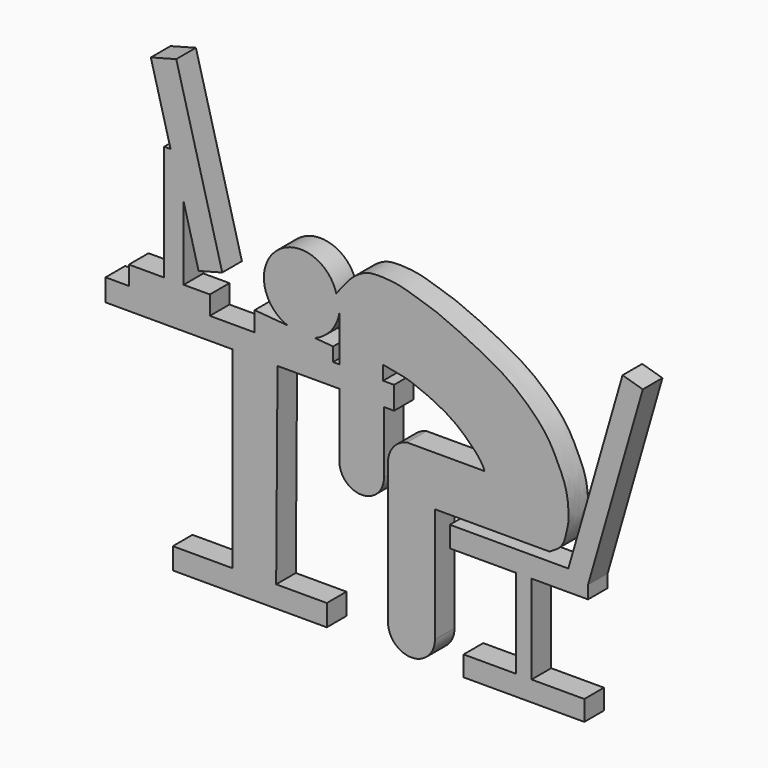
from build123d import *

# Parameters (mm, degrees)
F1_DEPTH = 2


# Not quite as in the source:
# - a feature of the source that left no trace in its solid (it failed there, or was rolled back) is left out


with BuildPart() as f1:
    # F0 (on Front) → F1 (new body)
    with BuildSketch(Plane.XZ):
        with BuildLine():
            Line((18.9171390745, 18.8327007444), (18.9171390745, 19.9865035199))
            add(Edge.make_bspline(
                [(18.9171390745, 19.9865035199), (20.2359017059, 19.7609265773), (20.9778353537, 19.6205597026), (23.2221259054, 18.699726427), (24.7231770067, 17.8086116304), (25.7698344015, 16.9044499376), (26.9919522107, 15.6755559146), (27.1760820528, 15.0417076929)],
                knots=[0, 0, 0, 0, 0.2179321827, 0.4264477532, 0.6140262018, 0.7851447158, 1, 1, 1, 1], degree=3))
            Line((27.1760820528, 15.0417076929), (20.8682008088, 15.0417076929))
            ThreePointArc((20.8682008088, 15.0417076929), (19.753969154, 14.3510608736), (19.318478182, 13.1145929918))
            Line((19.318478182, 13.1145929918), (19.318478182, 1.6501822975))
            ThreePointArc((19.318478182, 1.6501822975), (21.2292131037, -0.2605526242), (23.1399480253, 1.6501822975))
            Line((23.1399480253, 1.6501822975), (23.1399480253, 10.9915547073))
            Line((23.1399480253, 10.9915547073), (32.4813202024, 10.9915547073))
            add(Edge.make_bspline(
                [(32.4813202024, 10.9915547073), (32.7173913015, 11.1297281374), (33.1759580653, 11.3981287793), (33.6647764756, 11.943610763), (33.8785442051, 12.9474288042), (34.0688789671, 13.6968216831), (33.9783273465, 15.2441055836), (33.7191306214, 16.3712863899), (33.0805074051, 17.736024655), (32.5118657998, 18.8903594103), (31.6952000931, 19.9920483371), (30.3992394359, 21.2421100827), (29.0660577632, 22.3165505623), (27.023596623, 23.4836145379), (24.8210679729, 24.5125473654), (23.0257936504, 25.3081835207), (21.5598125958, 25.6984832194), (20.1925631903, 26.2037521602), (18.1718154029, 26.3052282349), (17.4545886694, 26.1074868938), (16.9452981604, 25.8397557796), (16.5052029261, 25.5141227487), (16.0173593733, 25.032961087), (15.6388983087, 24.5073680239), (15.2971428532, 24.1187135914), (15.2342961271, 24.0202073944), (15.1027834162, 23.8599643513)],
                knots=[0, 0, 0, 0, 0.0347440285, 0.0675998285, 0.1060000091, 0.1409634696, 0.1884405393, 0.2312071797, 0.278406367, 0.3225834899, 0.3679062968, 0.4197184745, 0.4708155203, 0.5303573368, 0.5916893616, 0.6460983797, 0.6931553162, 0.7409705446, 0.7957371438, 0.829037657, 0.8575649043, 0.886308658, 0.9185072385, 0.9504623164, 0.9766266121, 1, 1, 1, 1], degree=3))
            ThreePointArc((15.1027834162, 23.8599643513), (10.197746642, 25.3005876217), (11.1293799055, 20.2739743856))
            Line((11.1293799055, 20.2739743856), (8.4521435651, 20.4934416608))
            Line((8.4521435651, 20.4934416608), (8.4521435651, 18.8977912164))
            Line((8.4521435651, 18.8977912164), (4.807944844, 18.8977912164))
            Line((4.807944844, 18.8977912164), (4.807944844, 20.4323317588))
            Line((4.807944844, 20.4323317588), (2.6752410345, 20.4323317588))
            Line((2.6752410345, 20.4323317588), (2.6752410345, 26.3858548469))
            Line((2.6752410345, 26.3858548469), (3.8895721523, 21.8198716526))
            Line((3.8895721523, 21.8198716526), (5.8167126214, 22.3323979893))
            Line((5.8167126214, 22.3323979893), (2.0711510672, 36.4160123011))
            Line((2.0711510672, 36.4160123011), (0, 35.8651860971))
            Line((0, 35.8651860971), (1.6072647653, 29.8217406155))
            Line((1.6072647653, 29.8217406155), (1.0897519525, 29.8217406155))
            Line((1.0897519525, 29.8217406155), (1.0897519525, 20.4323317588))
            Line((1.0897519525, 20.4323317588), (-1.7866106892, 20.4323317588))
            Line((-1.7866106892, 20.4323317588), (-1.7866106892, 18.8977912164))
            Line((-1.7866106892, 18.8977912164), (-3.689032536, 18.8977912164))
            Line((-3.689032536, 18.8977912164), (-3.689032536, 17.0990628984))
            Line((-3.689032536, 17.0990628984), (6.6705888528, 17.0990628984))
            Line((6.6705888528, 17.0990628984), (6.6705888528, 1.4034443302))
            Line((6.6705888528, 1.4034443302), (1.7907759175, 1.4034443302))
            Line((1.7907759175, 1.4034443302), (1.7907759175, -0.3403924929))
            Line((1.7907759175, -0.3403924929), (14.3317757174, -0.3403924929))
            Line((14.3317757174, -0.3403924929), (14.3317757174, 1.4034443302))
            Line((14.3317757174, 1.4034443302), (10.2082798046, 1.4034443302))
            Line((10.2082798046, 1.4034443302), (10.3189582005, 17.0990628984))
            Line((10.3189582005, 17.0990628984), (15.356608129, 17.0990628984))
            Line((15.356608129, 17.0990628984), (15.356608129, 11.8973655189))
            ThreePointArc((15.356608129, 11.8973655189), (17.1713152045, 10.0826584434), (18.98602228, 11.8973655189))
            Line((18.98602228, 11.8973655189), (18.98602228, 16.9728393323))
            Line((18.98602228, 16.9728393323), (19.8126273521, 16.9728393323))
            Line((19.8126273521, 16.9728393323), (19.8126273521, 18.8327007444))
            Line((19.8126273521, 18.8327007444), (18.9171390745, 18.8327007444))
        make_face()
        with BuildLine():
            ThreePointArc((13.3592773256, 20.0911778564), (14.6775576036, 21.0436813613), (15.356608129, 22.5215230991))
            Line((15.356608129, 22.5215230991), (15.356608129, 18.8504233956))
            Line((15.356608129, 18.8504233956), (14.8478032858, 18.8504233956))
            Line((14.8478032858, 18.8504233956), (14.8478032858, 19.9691554815))
            Line((14.8478032858, 19.9691554815), (13.3592773256, 20.0911778564))
        make_face(mode=Mode.SUBTRACT)
    extrude(amount=F1_DEPTH)


with BuildPart() as f1b:
    # F0 (on Front) → F1, piece 2 (new body)
    with BuildSketch(Plane.XZ):
        Polygon((38.4207926691, 25.5733374506), (34.0049751103, 10.2760819718), (24.3503656238, 10.2760819718), (24.3503656238, 8.5804695264), (29.7309551388, 8.5804695264), (29.7309551388, 1.3424385106), (25.474363938, 1.3424385106), (25.474363938, -0.3008880303), (35.3066762154, -0.3008880303), (35.3066762154, 1.3424385106), (31.0113914311, 1.3424385106), (31.0113914311, 8.5804695264), (35.6110706925, 8.5804695264), (35.6110706925, 9.6396217123), (40.0729418852, 25.096415984), align=None)
    extrude(amount=F1_DEPTH)


solid = Compound([f1.part, f1b.part])
